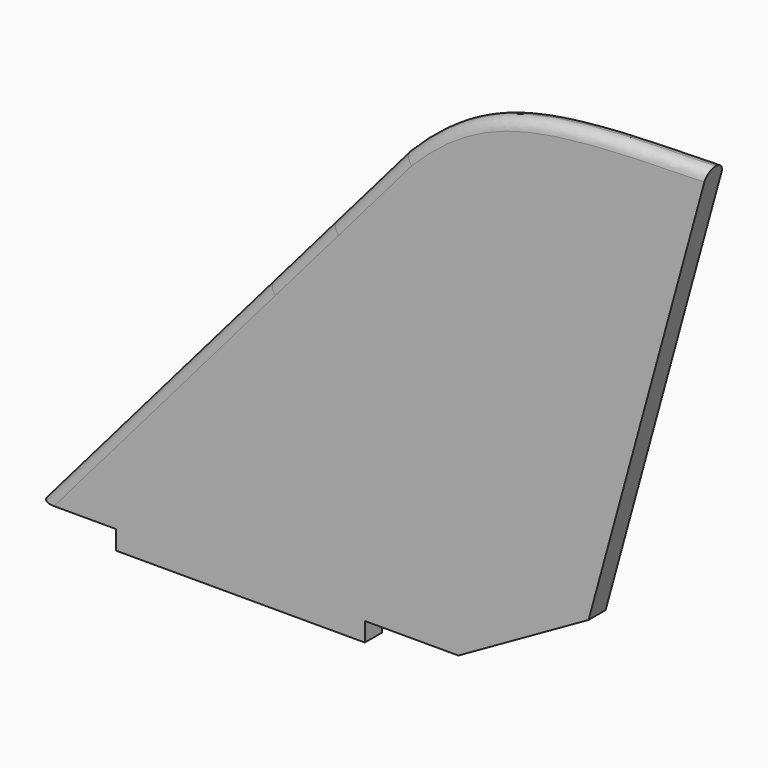
from build123d import *

# Parameters (mm, degrees)
F1_DEPTH = 2.8
F2_R     = 1.3999


# Not quite as in the source:
# - a fillet or chamfer is up to 0.001 mm smaller than in the source, because OpenCascade refuses the exact size
# - a feature names something its author has since deleted; it is built from what else it names


with BuildPart() as f1:
    # F0 (on Front) → F1 (new body)
    with BuildSketch(Plane.XZ):
        with BuildLine():
            Line((-25, -28.75), (7.7, -28.75))
            Line((7.7, -28.75), (7.7, -26.25))
            Line((7.7, -26.25), (20, -26.25))
            Line((20, -26.25), (37.1087677777, -16.5689531714))
            Line((37.1087677777, -16.5689531714), (52.7158603072, 40.4480434954))
            add(Edge.make_bspline(
                [(12.8214843672, 29.3465693193), (17.0304067433, 33.5662439466), (26.6575691876, 40.2533537434), (43.750764433, 40.2343917171), (52.7158603072, 40.4480434954)],
                knots=[0, 0, 0, 0, 0.4474896075, 1, 1, 1, 1], degree=3))
            Line((12.8214843672, 29.3465693193), (3.2140899724, 18.1771508975))
            Line((3.2140899724, 18.1771508975), (-5.0946967868, 8.517475019))
            Line((-5.0946967868, 8.517475019), (-35, -26.25))
            Line((-35, -26.25), (-25, -26.25))
            Line((-25, -26.25), (-25, -28.75))
        make_face()
    extrude(amount=F1_DEPTH)

    # F2 (radius 1.4 in the source; OpenCascade refuses exactly that, so slightly less here)
    f2_edges = [f1.edges().sort_by_distance(p)[0] for p in [
        (-11.089258, -2.8, 1.548285),
        (-11.089258, 0, 1.548285),
        (31.385103, -2.8, 39.151355),
        (31.385103, 0, 39.151355),
    ]]
    fillet(f2_edges, radius=F2_R)


solid = f1.part
